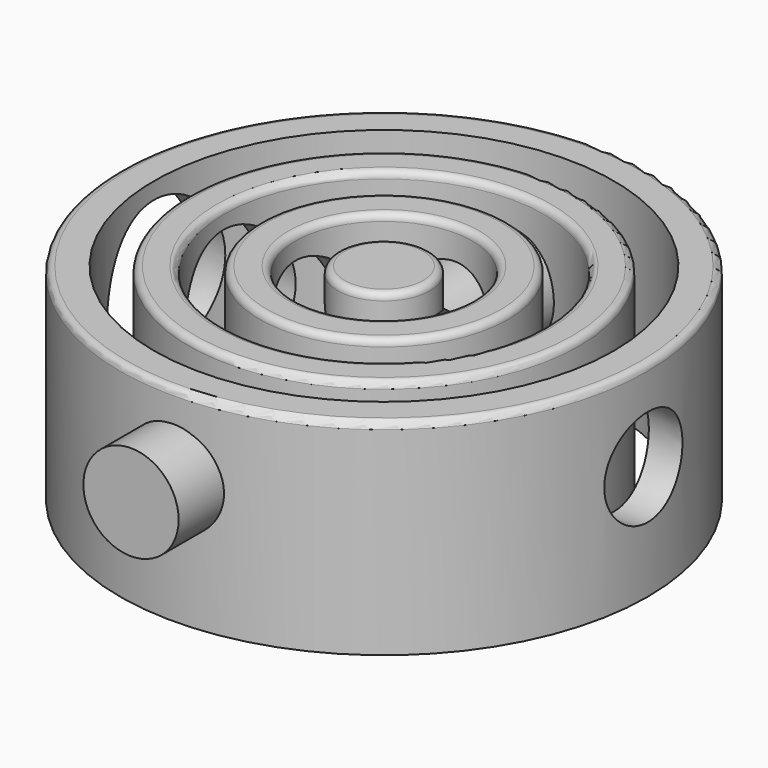
from build123d import *

# Parameters (mm, degrees)
F0_R          = 195.8548637347
F0_R_2        = 170.6264378578
F1_DEPTH      = 152.4
F0_R_3        = 34.3072775131
F0_R_4        = 92.1405938024
F0_R_5        = 65.6054553157
F0_R_6        = 145.1184649233
F0_R_7        = 119.0053222678
F2_R          = 5.08
F2_2_R        = 5.08
F2_3_R        = 5.08
F2_4_R        = 5.08
F4_R          = 35.3386545968
F5_DEPTH      = 457.2
F7_R          = 35.6870990296
F8_DEPTH      = 399.0558637347
F8_TAPER      = -3
F8_DEPTH_BACK = 159.6973240376


# Not quite as in the source:
# - the program builds the solid bodies; features that only make, move or delete a surface that nothing else refers to are left out


with BuildPart() as f1:
    # F0 (on Top) → F1 (new body)
    with BuildSketch(Plane.XY):
        Circle(F0_R)
        Circle(F0_R_2, mode=Mode.SUBTRACT)
    extrude(amount=F1_DEPTH)

    # F2
    f2_edges = [f1.edges().sort_by_distance(p)[0] for p in [
        (-195.854864, 0, 152.4),
    ]]
    fillet(f2_edges, radius=F2_R)


with BuildPart() as f1b:
    # F0 (on Top) → F1, piece 2 (new body)
    with BuildSketch(Plane.XY):
        Circle(F0_R_3)
    extrude(amount=F1_DEPTH)

    # F2#4
    f2_4_edges = [f1b.edges().sort_by_distance(p)[0] for p in [
        (-34.307278, 0, 152.4),
    ]]
    fillet(f2_4_edges, radius=F2_4_R)


with BuildPart() as f1c:
    # F0 (on Top) → F1, piece 3 (new body)
    with BuildSketch(Plane.XY):
        Circle(F0_R_4)
        Circle(F0_R_5, mode=Mode.SUBTRACT)
    extrude(amount=F1_DEPTH)

    # F2#3
    f2_3_edges = [f1c.edges().sort_by_distance(p)[0] for p in [
        (-92.140594, 0, 152.4),
        (-65.605455, 0, 152.4),
    ]]
    fillet(f2_3_edges, radius=F2_3_R)


with BuildPart() as f1d:
    # F0 (on Top) → F1, piece 4 (new body)
    with BuildSketch(Plane.XY):
        Circle(F0_R_6)
        Circle(F0_R_7, mode=Mode.SUBTRACT)
    extrude(amount=F1_DEPTH)

    # F2#2
    f2_2_edges = [f1d.edges().sort_by_distance(p)[0] for p in [
        (-145.118465, 0, 152.4),
        (-119.005322, 0, 152.4),
    ]]
    fillet(f2_2_edges, radius=F2_2_R)


with BuildPart() as f5:
    # F4 (on offset) → F5 (new body)
    with BuildSketch(Plane.XZ.offset(234.6243560314)):
        with Locations((0, 93.4201031923)):
            Circle(F4_R)
    extrude(amount=-F5_DEPTH)


with BuildPart() as f8_tool:
    # F7 (on offset) → F8 (new body, two sides)
    with BuildSketch(Plane.YZ.offset(203.2)) as f8_sk:
        with Locations((0, 84.7620144486)):
            Circle(F7_R)
    extrude(amount=-F8_DEPTH, taper=F8_TAPER)
    extrude(f8_sk.sketch, amount=F8_DEPTH_BACK)


with BuildPart() as f1_1:
    add(f1.part)

    # F8: cut by f8_tool
    add(f8_tool.part, mode=Mode.SUBTRACT)


with BuildPart() as f1b_1:
    add(f1b.part)

    # F8: cut by f8_tool
    add(f8_tool.part, mode=Mode.SUBTRACT)


with BuildPart() as f1c_1:
    add(f1c.part)

    # F8: cut by f8_tool
    add(f8_tool.part, mode=Mode.SUBTRACT)


with BuildPart() as f1d_1:
    add(f1d.part)

    # F8: cut by f8_tool
    add(f8_tool.part, mode=Mode.SUBTRACT)


with BuildPart() as f5_1:
    add(f5.part)

    # F8: cut by f8_tool
    add(f8_tool.part, mode=Mode.SUBTRACT)


solid = Compound([f1_1.part, f1b_1.part, f1c_1.part, f1d_1.part, f5_1.part])
